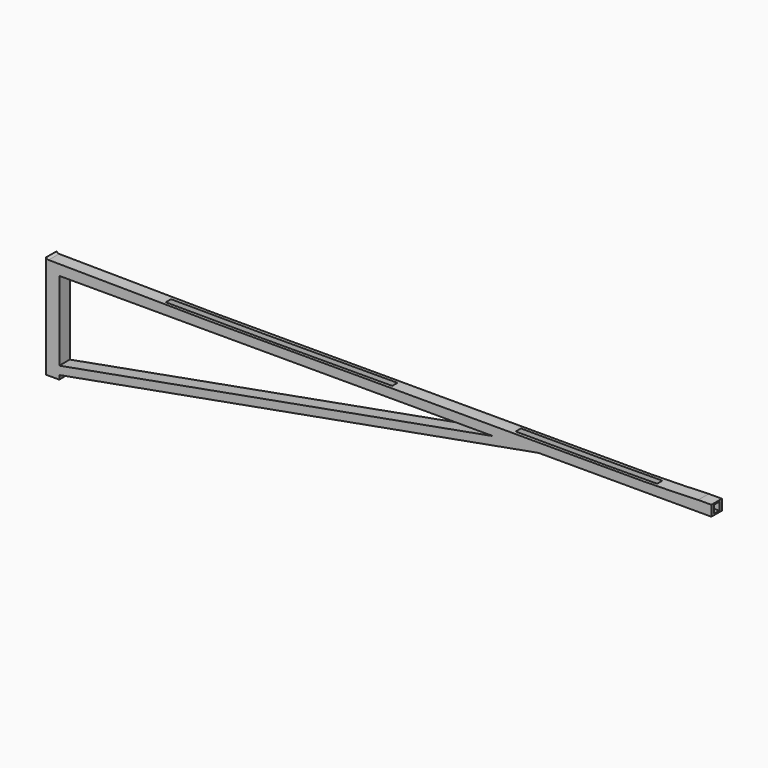
from build123d import *

# Parameters (mm, degrees)
F1_DEPTH = 10
F2_W     = 5
F2_H     = 6
F3_DEPTH = 495
F4_W     = 10
F4_H     = 10.6507557631
F5_DEPTH = 25


with BuildPart() as f1:
    # F0 (on Front) → F1 (new body)
    with BuildSketch(Plane.XZ):
        with BuildLine():
            Line((0, 8), (0, 0))
            Line((0, 0), (0, -80))
            Line((0, -80), (10, -80))
            Line((10, -80), (10, -66.2595003911))
            Line((10, -66.2595003911), (373.7241029739, 0))
            Line((373.7241029739, 0), (505, 0))
            Line((505, 0), (505, 8))
            Line((505, 8), (495, 8))
            add(Edge.make_bspline(
                [(1.8815460355, 7.9757237206), (41.9158968697, 7.4592539668), (121.7303576786, 6.4418774159), (248.8795131648, 6.9843016), (337.5487991179, 7.2325436144), (457.5810815868, 6.3868246941), (483.8835547527, 7.5984463681), (495, 8)],
                knots=[0.0035028054, 0.0035028054, 0.0035028054, 0.0035028054, 0.2271440961, 0.4556460712, 0.6558474221, 0.8763222147, 1, 1, 1, 1], degree=3))
            add(Edge.make_bspline(
                [(0, 8), (0.627325076, 7.9919054957), (1.2545037706, 7.9838129829), (1.8815460355, 7.9757237206)],
                knots=[0, 0, 0, 0, 0.0035028054, 0.0035028054, 0.0035028054, 0.0035028054], degree=3))
        make_face()
        Polygon((10, -60), (10, 0), (339.3632769585, 0), align=None, mode=Mode.SUBTRACT)
        with BuildLine():
            Line((0, 9.1209262609), (0, 8))
            add(Edge.make_bspline(
                [(0, 8), (0.627325076, 7.9919054957), (1.2545037706, 7.9838129829), (1.8815460355, 7.9757237206)],
                knots=[0, 0, 0, 0, 0.0035028054, 0.0035028054, 0.0035028054, 0.0035028054], degree=3))
            add(Edge.make_bspline(
                [(1.8815460355, 7.9757237206), (1.4466139308, 8.041002586), (0.6078738326, 8.1668889057), (0.1975491446, 8.8108795813), (0, 9.1209262609)],
                knots=[0, 0, 0, 0, 0.5185540858, 1, 1, 1, 1], degree=3))
        make_face()
    extrude(amount=F1_DEPTH)

    # F2 (on face) → F3 (cut)
    with BuildSketch(Plane.YZ.offset(505)):
        with Locations((-5, 4)):
            Rectangle(F2_W, F2_H)
    extrude(amount=-F3_DEPTH, mode=Mode.SUBTRACT)

    # F4 (on face) → F5 (cut)
    with BuildSketch(Plane.XZ.offset(10)):
        with Locations((5, -74.6746221185)):
            Rectangle(F4_W, F4_H)
    extrude(amount=-F5_DEPTH, mode=Mode.SUBTRACT)


solid = f1.part
